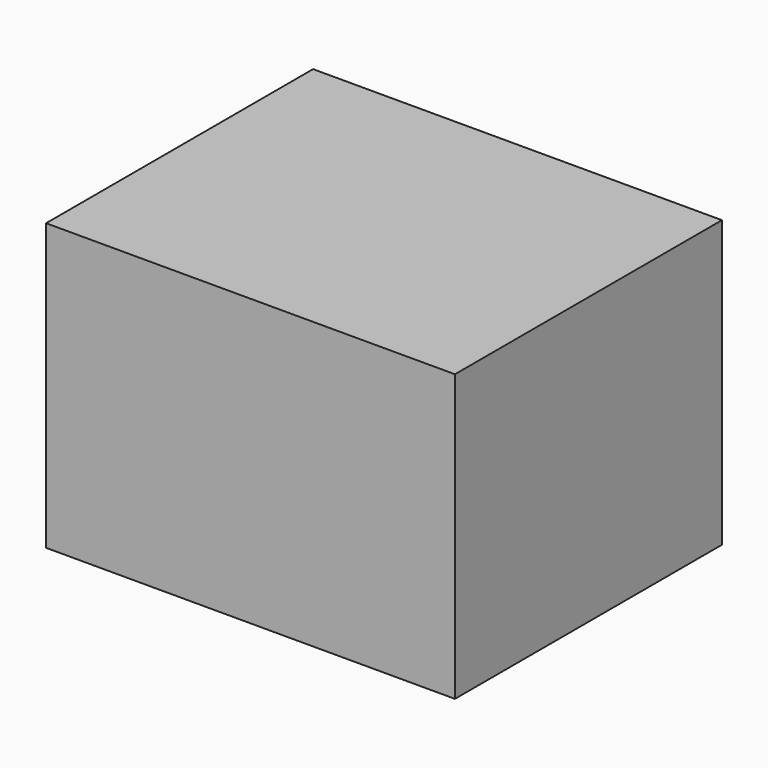
from build123d import *

# Parameters (mm, degrees)
F0_W     = 181.6942822188
F0_H     = 148.2967324555
F1_DEPTH = 127


with BuildPart() as f1:
    # F0 (on Top) → F1 (new body)
    with BuildSketch(Plane.XY):
        with Locations((-62.7455348149, -38.2277201861)):
            Rectangle(F0_W, F0_H)
    extrude(amount=F1_DEPTH)


solid = f1.part
